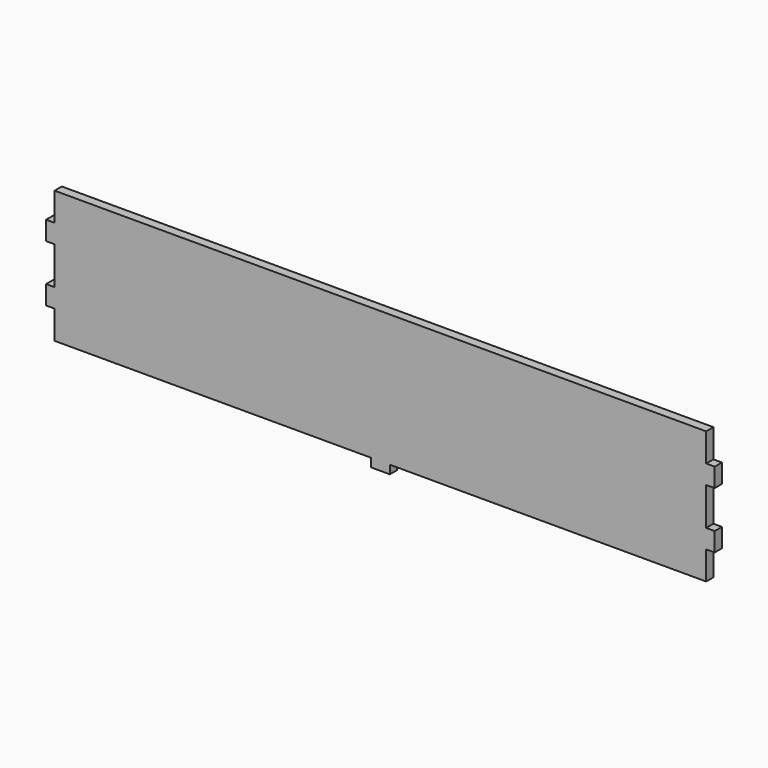
from build123d import *

# Parameters (mm, degrees)
F0_W     = 4.5
F0_H     = 10
F1_DEPTH = 4.8


# Not quite as in the source:
# - a feature names something its author has since deleted; it is built from what else it names


with BuildPart() as f1:
    # F0 (on Front) → F1 (new body)
    with BuildSketch(Plane.XZ):
        Polygon((-167.476225, 0), (0, 0), (0, 15), (4.5, 15), (4.5, 25), (0, 25), (0, 45), (4.5, 45), (4.5, 55), (0, 55), (0, 70), (-172.276225, 70), (-182.276225, 70), (-344.95245, 70), (-344.95245, 55), (-349.45245, 55), (-349.45245, 45), (-344.95245, 45), (-344.95245, 25), (-344.95245, 15), (-344.95245, 0), (-177.476225, 0), align=None)
        Polygon((-167.476225, -0.2312080078), (-167.476225, 0), (-177.476225, 0), (-177.476225, -4.5), (-167.476225, -4.5), align=None)
        with Locations((-347.20245, 20)):
            Rectangle(F0_W, F0_H)
    extrude(amount=F1_DEPTH)


solid = f1.part
